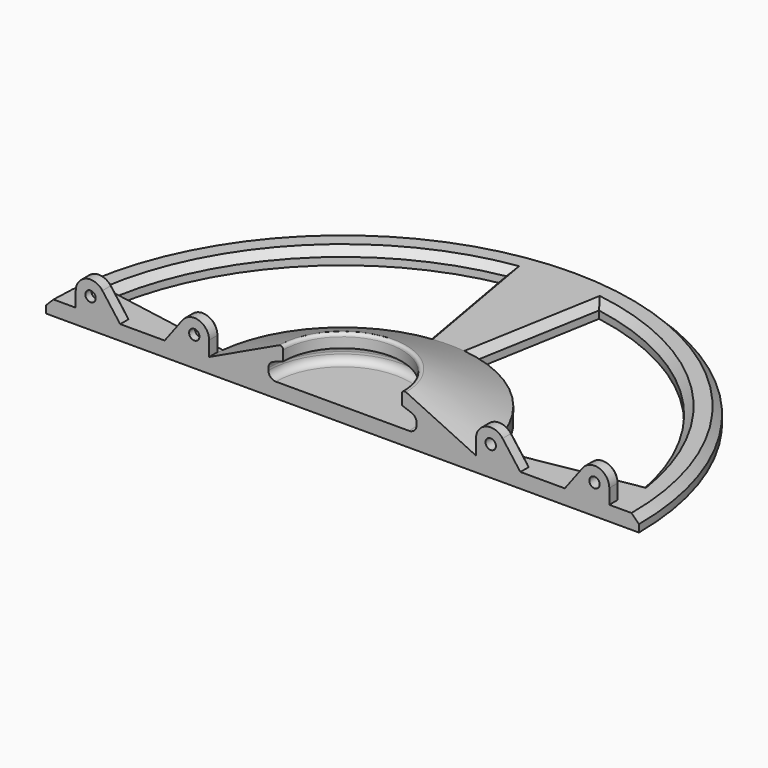
from build123d import *

# Parameters (mm, degrees)
F1_ANGLE      = 180
F0_W          = 10
F0_H          = 5
F2_R          = 1
F3_R          = 2.5
F4_W          = 45
F4_H          = 5
F5_ANGLE      = 10
F6_W          = 45
F6_H          = 5
F7_ANGLE      = 10
F8_W          = 45
F8_H          = 5
F9_ANGLE_BACK = 10
F9_ANGLE      = 20
F10_R         = 1.75
F11_DEPTH     = 5
F13_DEPTH     = 2.5
F14_SIZE      = 2.5
F16_DEPTH     = 5
F17_SIZE      = 1.5


with BuildPart() as f1:
    # F0 (on Front) → F1 (revolve)
    with BuildSketch(Plane.XZ):
        Polygon((25, 0), (0, 0), (0, -5), (45, -5), (45, 0), (20, 11.8198511713), (20, 6.8198511713), (25, 5), align=None)
    revolve(axis=Axis((0, 0, -2.5), (0, 0, 1)), revolution_arc=F1_ANGLE)

    # F2
    f2_edges = [f1.edges().sort_by_distance(p)[0] for p in [
        (0, 20, 11.819851),
    ]]
    fillet(f2_edges, radius=F2_R)

    # F3
    f3_edges = [f1.edges().sort_by_distance(p)[0] for p in [
        (0, 25, 5),
        (0, 25, 0),
    ]]
    fillet(f3_edges, radius=F3_R)



with BuildPart() as f1b:
    # F0 (on Front) → F1, piece 2 (revolve)
    with BuildSketch(Plane.XZ):
        with Locations((95, -2.5)):
            Rectangle(F0_W, F0_H)
    revolve(axis=Axis((0, 0, -2.5), (0, 0, 1)), revolution_arc=F1_ANGLE)


with BuildPart() as f1_1:
    add(f1.part)

    add(f1b.part)  # F5 merges F1b
    # F4 (on face) → F5 (revolve)
    with BuildSketch(Plane.XZ):
        with Locations((67.5, -2.5)):
            Rectangle(F4_W, F4_H)
    revolve(axis=Axis((0, 0, 10), (0, 0, 1)), revolution_arc=F5_ANGLE)

    # F6 (on face) → F7 (revolve)
    with BuildSketch(Plane.XZ):
        with Locations((-67.5, -2.5)):
            Rectangle(F6_W, F6_H)
    revolve(axis=Axis((0, 0, 10), (0, 0, -1)), revolution_arc=F7_ANGLE)

    # F8 (on Right) → F9 (revolve)
    with BuildSketch(Plane.YZ, mode=Mode.PRIVATE) as f9_sk:
        with Locations((67.5, -2.5)):
            Rectangle(F8_W, F8_H)
    revolve(f9_sk.sketch.rotate(Axis((0, 0, 10), (0, 0, 1)), -F9_ANGLE_BACK), axis=Axis((0, 0, 10), (0, 0, 1)), revolution_arc=F9_ANGLE)

    # F10 (on face) → F11 (join)
    with BuildSketch(Plane.XZ):
        with BuildLine():
            Line((-90, 5), (-90, 0))
            Line((-90, 0), (-80, 0))
            Line((-80, 0), (-80, 5))
            ThreePointArc((-80, 5), (-85, 10), (-90, 5))
        make_face()
        with Locations((-85, 5)):
            Circle(F10_R, mode=Mode.SUBTRACT)
        with BuildLine():
            Line((-55, 0), (-45, 0))
            Line((-45, 0), (-45, 5))
            ThreePointArc((-45, 5), (-50, 10), (-55, 5))
            Line((-55, 5), (-55, 0))
        make_face()
        with Locations((-50, 5)):
            Circle(F10_R, mode=Mode.SUBTRACT)
        with BuildLine():
            Line((80, 5), (80, 0))
            Line((80, 0), (90, 0))
            Line((90, 0), (90, 5))
            ThreePointArc((90, 5), (85, 10), (80, 5))
        make_face()
        with Locations((85, 5)):
            Circle(F10_R, mode=Mode.SUBTRACT)
        with BuildLine():
            Line((45, 0), (55, 0))
            Line((55, 0), (55, 5))
            ThreePointArc((55, 5), (50, 10), (45, 5))
            Line((45, 5), (45, 0))
        make_face()
        with Locations((50, 5)):
            Circle(F10_R, mode=Mode.SUBTRACT)
    extrude(amount=-F11_DEPTH)

    # F12 (on face) → F13 (cut)
    with BuildSketch(Plane(origin=(0, 5, 0), x_dir=(-1, 0, 0), z_dir=(0, 1, 0))):
        Polygon((52.75, 3.4122867597), (52.75, 6.5877132403), (50, 8.1754264805), (47.25, 6.5877132403), (47.25, 3.4122867597), (50, 1.8245735195), align=None)
        Polygon((82.25, 6.5877132403), (82.25, 3.4122867597), (85, 1.8245735195), (87.75, 3.4122867597), (87.75, 6.5877132403), (85, 8.1754264805), align=None)
    extrude(amount=-F13_DEPTH, mode=Mode.SUBTRACT)

    # F14
    f14_edges = [f1_1.edges().sort_by_distance(p)[0] for p in [
        (-11.721252, 66.474523, 0),
        (11.721252, 66.474523, 0),
        (-63.63961, 63.63961, 0),
        (-66.474523, 11.721252, 0),
        (66.474523, 11.721252, 0),
        (63.63961, 63.63961, 0),
        (0, 100, 0),
    ]]
    chamfer(f14_edges, length=F14_SIZE)

    # F15 (on face) → F16 (join, through all)
    with BuildSketch(Plane.XZ):
        with BuildLine():
            Line((-80, 0), (-75, 0))
            Line((-75, 0), (-81, 8))
            ThreePointArc((-81, 8), (-80.2565835097, 6.5811388301), (-80, 5))
            Line((-80, 5), (-80, 0))
        make_face()
        with BuildLine():
            Line((-60, 0), (-55, 0))
            Line((-55, 0), (-55, 5))
            ThreePointArc((-55, 5), (-54.7434164903, 6.5811388301), (-54, 8))
            Line((-54, 8), (-60, 0))
        make_face()
        with BuildLine():
            ThreePointArc((54, 8), (54.7434164903, 6.5811388301), (55, 5))
            Line((55, 5), (55, 0))
            Line((55, 0), (60, 0))
            Line((60, 0), (54, 8))
        make_face()
        with BuildLine():
            Line((80, 0), (80, 5))
            ThreePointArc((80, 5), (80.2565835097, 6.5811388301), (81, 8))
            Line((81, 8), (75, 0))
            Line((75, 0), (80, 0))
        make_face()
    extrude(amount=-F16_DEPTH)

    # F17
    f17_edges = [f1_1.edges().sort_by_distance(p)[0] for p in [
        (-57, 5, 4),
        (-78, 5, 4),
        (78, 5, 4),
        (57, 5, 4),
        (90, 5, 2.5),
        (86.581139, 5, 9.743416),
        (48.418861, 5, 9.743416),
        (45, 5, 2.5),
        (-45, 5, 2.5),
        (-48.418861, 5, 9.743416),
        (-86.581139, 5, 9.743416),
        (-90, 5, 2.5),
    ]]
    chamfer(f17_edges, length=F17_SIZE)


solid = f1_1.part
